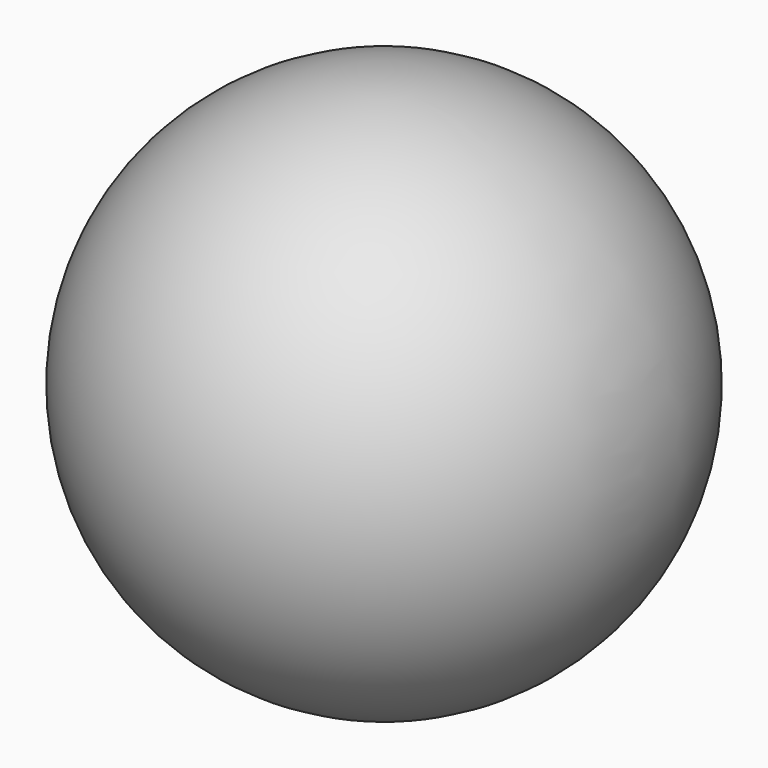
from build123d import *


# Not quite as in the source:
# - a feature names something its author has since deleted; it is built from what else it names


with BuildPart() as f1:
    # F0 (on Front) → F1 (revolve)
    with BuildSketch(Plane.XZ):
        with BuildLine():
            ThreePointArc((0, -500), (353.5533905933, -353.5533905933), (500, 0))
            ThreePointArc((500, 0), (353.5533905933, 353.5533905933), (0, 500))
            Line((0, 500), (0, -500))
        make_face()
    revolve(axis=Axis((0, 0, 0), (0, 0, -1)))


solid = f1.part
